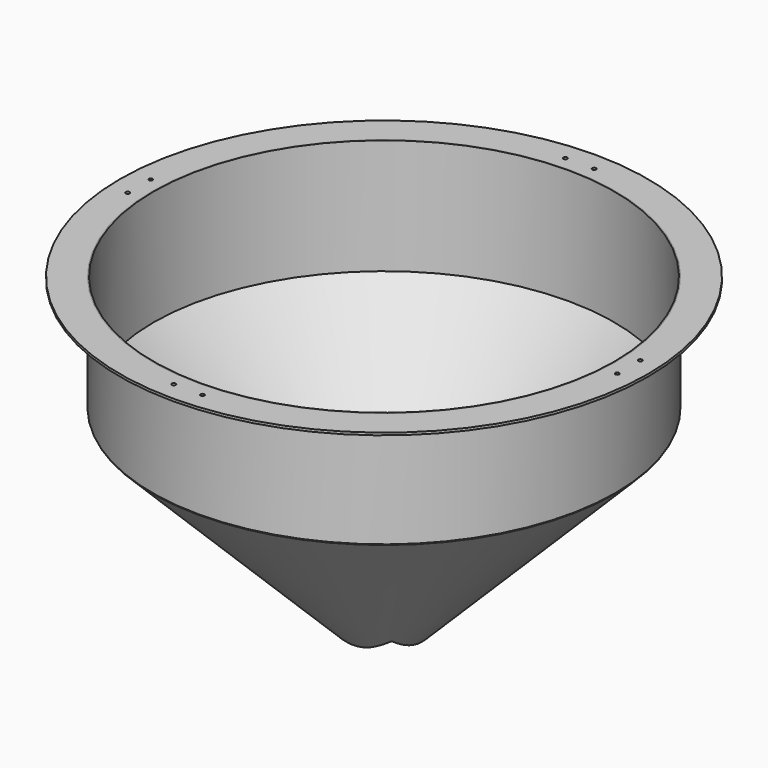
from build123d import *

# Parameters (mm, degrees)
F2_W            = 203.2
F2_H            = 203.2
F3_DEPTH        = 2.2460640303
F3_DEPTH_BACK   = 609.601
F4_W            = 3.175
F4_H            = 304.8
F6_W            = 85.725
F6_H            = 6.35
F9_D            = 10.31875
F9_COPIES_COUNT = 4


# Not quite as in the source:
# - a length typed as a fraction of an inch, garbled in the dataset ("3 / 203.2 mm" for 3/8 in), is restored
# - a pattern or mirror of a feature is missing from the dataset's text; its kind, count and spacing are read off the source's solid


with BuildPart() as f1:
    # F0 (on Front) → F1 (revolve)
    with BuildSketch(Plane.XZ):
        Polygon((609.6, 609.6), (2.2450640303, 2.2450640303), (2.2450640303, -2.2450640303), (611.8450640303, 607.3549359697), align=None)
    revolve(axis=Axis((0, 0, 23.5767196864), (0, 0, 1)))

    # F2 (on Top) → F3 (cut, two sides)
    with BuildSketch(Plane.XY) as f3_sk:
        Rectangle(F2_W, F2_H)
    extrude(amount=-F3_DEPTH, mode=Mode.SUBTRACT)
    extrude(f3_sk.sketch, amount=F3_DEPTH_BACK, mode=Mode.SUBTRACT)


with BuildPart() as f5:
    # F4 (on Front) → F5 (revolve)
    with BuildSketch(Plane.XZ):
        with Locations((611.1875, 762)):
            Rectangle(F4_W, F4_H)
    revolve(axis=Axis((0, 0, 23.5767196864), (0, 0, 1)))


with BuildPart() as f7:
    # F6 (on Front) → F7 (revolve)
    with BuildSketch(Plane.XZ):
        with Locations((655.6375, 911.225)):
            Rectangle(F6_W, F6_H)
    revolve(axis=Axis((0, 0, 23.5767196864), (0, 0, 1)))

    # F9 (through all)
    with Locations(Plane.XY.offset(914.4)):
        with Locations((647.7, 38.1), (647.7, -38.1)):
            f9 = Hole(F9_D / 2)

    # F9_copies: F9 ×4 about axis
    f9_copies_axis = Axis((0, 0, 0), (0, 0, 1))
    for i in range(1, F9_COPIES_COUNT):
        add(f9.rotate(f9_copies_axis, i * 360 / F9_COPIES_COUNT), mode=Mode.SUBTRACT)


solid = Compound([f1.part, f5.part, f7.part])
